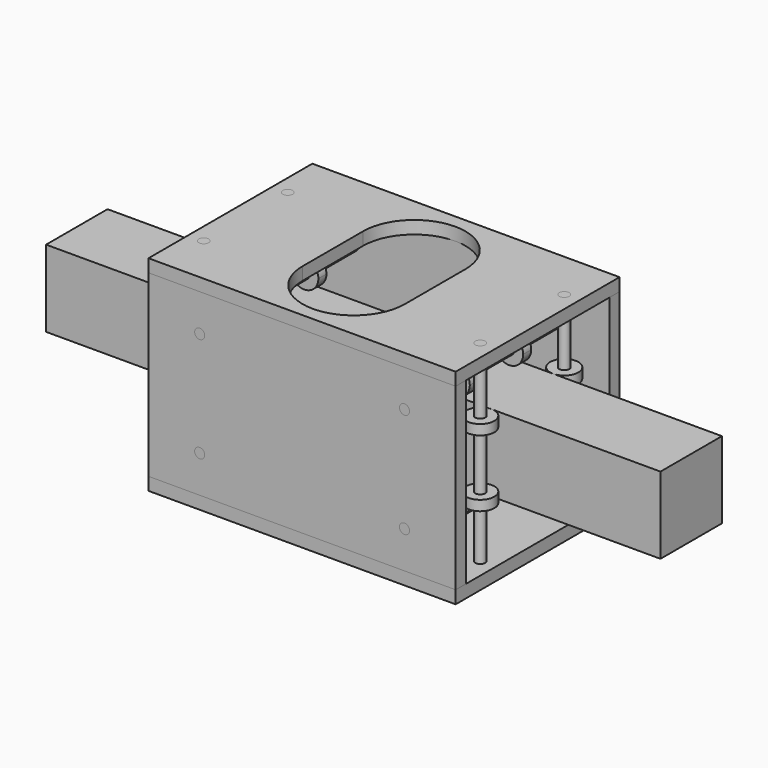
from build123d import *

# Parameters (mm, degrees)
F0_W      = 304.8
F0_H      = 38.1
F1_DEPTH  = 19.05
F2_R      = 2.5
F3_DEPTH  = 5
F6_R      = 2.5
F7_DEPTH  = 50.8
F10_W     = 152.4
F10_H     = 88.9
F10_R     = 2.5
F11_DEPTH = 6.35
F13_W     = 152.4
F13_H     = 95.25
F13_H_2   = 6.35
F14_DEPTH = 6.35
F15_R     = 2.5
F16_DEPTH = 5
F20_R     = 2.5
F21_DEPTH = 6.35
F23_R     = 2.5
F24_DEPTH = 101.6


with BuildPart() as f1:
    # F0 (on Front) → F1 (new body, symmetric)
    with BuildSketch(Plane.XZ):
        Rectangle(F0_W, F0_H)
    extrude(amount=F1_DEPTH, both=True)


with BuildPart() as f3:
    # F2 (on face) → F3 (new body)
    with BuildSketch(Plane.XZ.offset(19.05)):
        with BuildLine():
            ThreePointArc((-50.8, 19.0499995202), (-45.8502525317, 21.1002520519), (-43.8, 26.0499995202))
            ThreePointArc((-43.8, 26.0499995202), (-55.7497474683, 30.9997469885), (-50.8, 19.0499995202))
        make_face()
        with Locations((-50.8, 26.0499995202)):
            Circle(F2_R, mode=Mode.SUBTRACT)
    extrude(amount=-F3_DEPTH)


with BuildPart() as f3b:
    # F2 (on face) → F3, piece 2 (new body)
    with BuildSketch(Plane.XZ.offset(19.05)):
        with BuildLine():
            ThreePointArc((57.8000012957, 26.0500012957), (45.8502516313, 30.9997496959), (50.7999999553, 19.05))
            ThreePointArc((50.7999999553, 19.05), (55.7497483687, 21.1002528954), (57.8000012957, 26.0500012957))
        make_face()
        with Locations((50.8, 26.0500012957)):
            Circle(F2_R, mode=Mode.SUBTRACT)
    extrude(amount=-F3_DEPTH)


with BuildPart() as f4_1:
    # F4: instance of F3
    add(f3.part.mirror(Plane.XZ))


with BuildPart() as f4_2:
    # F4: instance of F3b
    add(f3b.part.mirror(Plane.XZ))


with BuildPart() as f5_1:
    # F5: instance of F3b
    add(f3b.part.mirror(Plane.XY))


with BuildPart() as f5_2:
    # F5: instance of F4_2
    add(f4_2.part.mirror(Plane.XY))


with BuildPart() as f5_3:
    # F5: instance of F3
    add(f3.part.mirror(Plane.XY))


with BuildPart() as f5_4:
    # F5: instance of F4_1
    add(f4_1.part.mirror(Plane.XY))


with BuildPart() as f7:
    # F6 (on Front) → F7 (new body, symmetric)
    with BuildSketch(Plane.XZ):
        with Locations((-50.8, 26.0499995202)):
            Circle(F6_R)
    extrude(amount=F7_DEPTH, both=True)


with BuildPart() as f8_1:
    # F8: instance of F7
    add(f7.part.mirror(Plane.YZ))


with BuildPart() as f9_1:
    # F9: instance of F8_1
    add(f8_1.part.mirror(Plane.XY))


with BuildPart() as f9_2:
    # F9: instance of F7
    add(f7.part.mirror(Plane.XY))


with BuildPart() as f11:
    # F10 (on face) → F11 (new body)
    with BuildSketch(Plane.XZ.offset(50.8)):
        Rectangle(F10_W, F10_H)
        with Locations((-50.8, -26.0499995202)):
            Circle(F10_R, mode=Mode.SUBTRACT)
        with Locations((50.8, -26.0499995202)):
            Circle(F10_R, mode=Mode.SUBTRACT)
        with Locations((-50.8, 26.0499995202)):
            Circle(F10_R, mode=Mode.SUBTRACT)
        with Locations((50.8, 26.0499995202)):
            Circle(F10_R, mode=Mode.SUBTRACT)
    extrude(amount=-F11_DEPTH)


with BuildPart() as f12_1:
    # F12: instance of F11
    add(f11.part.mirror(Plane.XZ))


with BuildPart() as f14:
    # F13 (on face) → F14 (new body)
    with BuildSketch(Plane.XY.offset(44.45)):
        with Locations((0, -3.175)):
            Rectangle(F13_W, F13_H)
        with BuildLine():
            Line((-25.4, -18.7701191753), (-25.4, 18.7701191753))
            ThreePointArc((-25.4, 18.7701191753), (0, 44.1701191753), (25.4, 18.7701191753))
            Line((25.4, 18.7701191753), (25.4, -18.7701191753))
            ThreePointArc((25.4, -18.7701191753), (0, -44.1701191753), (-25.4, -18.7701191753))
        make_face(mode=Mode.SUBTRACT)
        with Locations((0, 47.625)):
            Rectangle(F13_W, F13_H_2)
    extrude(amount=F14_DEPTH)

    # F20 (on face) → F21 (cut, through all)
    with BuildSketch(Plane.XY.offset(50.8)):
        with Locations((-68.58, 26.05)):
            Circle(F20_R)
        with Locations((-68.58, -26.05)):
            Circle(F20_R)
        with Locations((68.58, 26.05)):
            Circle(F20_R)
        with Locations((68.58, -26.05)):
            Circle(F20_R)
    extrude(amount=-F21_DEPTH, mode=Mode.SUBTRACT)


with BuildPart() as f16:
    # F15 (on face) → F16 (new body)
    with BuildSketch(Plane.XY.offset(19.05)):
        with BuildLine():
            ThreePointArc((-68.58, 19.05), (-63.6302525317, 21.1002525317), (-61.58, 26.05))
            ThreePointArc((-61.58, 26.05), (-73.5297474683, 30.9997474683), (-68.58, 19.05))
        make_face()
        with Locations((-68.58, 26.05)):
            Circle(F15_R, mode=Mode.SUBTRACT)
    extrude(amount=-F16_DEPTH)


with BuildPart() as f17_1:
    # F17: instance of F16
    add(f16.part.mirror(Plane.XY))


with BuildPart() as f18_1:
    # F18: instance of F17_1
    add(f17_1.part.mirror(Plane.YZ))


with BuildPart() as f18_2:
    # F18: instance of F16
    add(f16.part.mirror(Plane.YZ))


with BuildPart() as f19_1:
    # F19: instance of F17_1
    add(f17_1.part.mirror(Plane.XZ))


with BuildPart() as f19_2:
    # F19: instance of F16
    add(f16.part.mirror(Plane.XZ))


with BuildPart() as f19_3:
    # F19: instance of F18_1
    add(f18_1.part.mirror(Plane.XZ))


with BuildPart() as f19_4:
    # F19: instance of F18_2
    add(f18_2.part.mirror(Plane.XZ))


with BuildPart() as f22_1:
    # F22: instance of F14
    add(f14.part.mirror(Plane.XY))


with BuildPart() as f24:
    # F23 (on face) → F24 (new body, through all)
    with BuildSketch(Plane.XY.offset(50.8)):
        with Locations((-68.58, 26.05)):
            Circle(F23_R)
    extrude(amount=-F24_DEPTH)


with BuildPart() as f24b:
    # F23 (on face) → F24, piece 2 (new body, through all)
    with BuildSketch(Plane.XY.offset(50.8)):
        with Locations((-68.58, -26.05)):
            Circle(F23_R)
    extrude(amount=-F24_DEPTH)


with BuildPart() as f24c:
    # F23 (on face) → F24, piece 3 (new body, through all)
    with BuildSketch(Plane.XY.offset(50.8)):
        with Locations((68.58, -26.05)):
            Circle(F23_R)
    extrude(amount=-F24_DEPTH)


with BuildPart() as f24d:
    # F23 (on face) → F24, piece 4 (new body, through all)
    with BuildSketch(Plane.XY.offset(50.8)):
        with Locations((68.58, 26.05)):
            Circle(F23_R)
    extrude(amount=-F24_DEPTH)


solid = Compound([f1.part, f3.part, f3b.part, f4_1.part, f4_2.part, f5_1.part, f5_2.part, f5_3.part, f5_4.part, f7.part, f8_1.part, f9_1.part, f9_2.part, f11.part, f12_1.part, f14.part, f16.part, f17_1.part, f18_1.part, f18_2.part, f19_1.part, f19_2.part, f19_3.part, f19_4.part, f22_1.part, f24.part, f24b.part, f24c.part, f24d.part])
